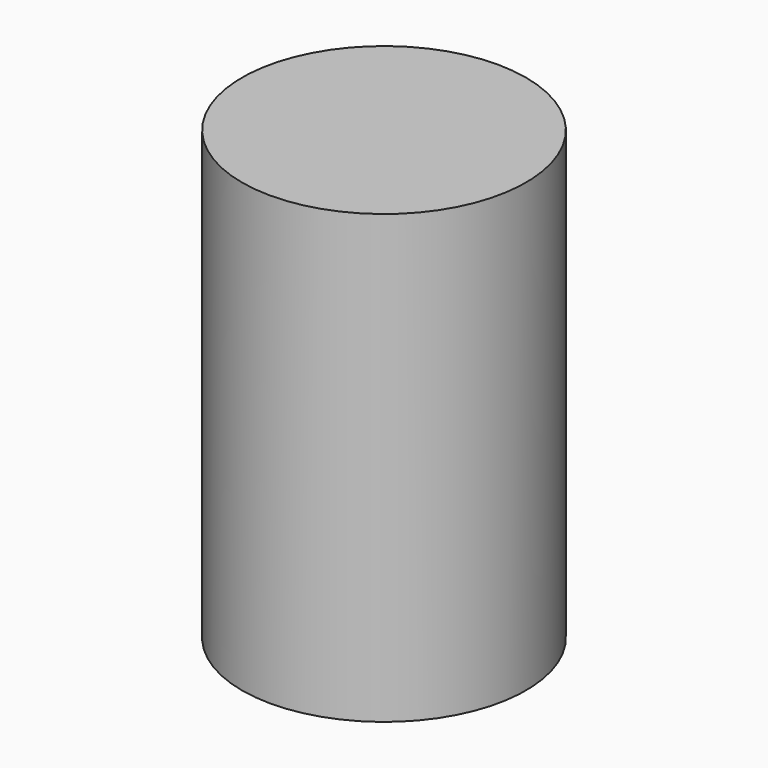
from build123d import *

# Parameters (mm, degrees)
F2_W = 5.4483478889
F2_H = 17.1522088349


# Not quite as in the source:
# - a feature of the source that left no trace in its solid (it failed there, or was rolled back) is left out


with BuildPart() as f3:
    # F2 (on Right) → F3 (revolve)
    with BuildSketch(Plane.YZ):
        with Locations((2.7241739444, 47.4208090454)):
            Rectangle(F2_W, F2_H)
    revolve(axis=Axis((0, 0, 47.4208090454), (0, 0, 1)))


solid = f3.part
